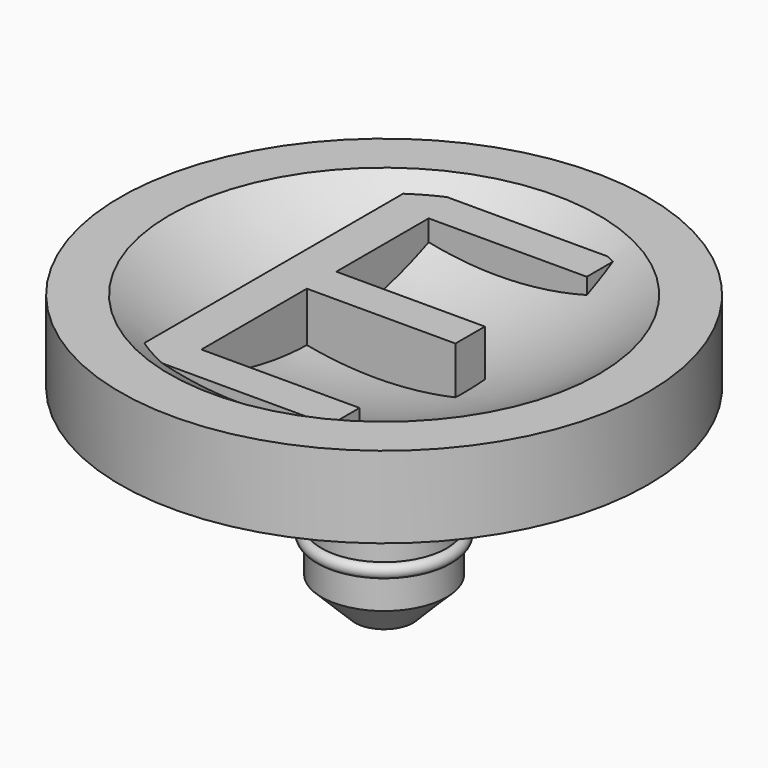
from build123d import *

# Parameters (mm, degrees)
F2_TEXT_SIZE = 19.0165314254
F3_DEPTH     = 3.4036
F4_W         = 439.3387079644
F4_H         = 117.3384692084
F5_DEPTH     = 12.7
F6_SIZE      = 1.27
F7_R         = 14.2800405429
F7_R_2       = 10
F7_R_3       = 5.842
F8_DEPTH     = 0.8
F9_SIZE      = 0.508


# Not quite as in the source:
# - Text() gives the source's letters only with a copy of the font that has no kerning and outlines rounded to 1/6400 em; it was checked with that copy


with BuildPart() as f1:
    # F0 (on Front) → F1 (revolve)
    with BuildSketch(Plane.XZ):
        with BuildLine():
            Line((2.6757909362, 0), (4.2185683136, 0))
            Line((4.2185683136, 0), (10, 0))
            Line((10, 0), (10, 5.4849551513))
            ThreePointArc((10, 5.4849551513), (5.4259986852, 2.3667937844), (0, 1.27))
            Line((0, 1.27), (0, 0))
            Line((0, 0), (0, -6.7))
            Line((0, -6.7), (2.3710267587, -6.7))
            Line((2.3710267587, -6.7), (2.3710267587, -4.308))
            ThreePointArc((2.3710267587, -4.308), (2.6250267587, -4.054), (2.3710267587, -3.8))
            Line((2.3710267587, -3.8), (2.3710267587, 0))
            Line((2.3710267587, 0), (2.6757909362, 0))
        make_face()
    revolve(axis=Axis((0, 0, 0.635), (0, 0, -1)))

    # F2 (on Top) → F3 (join)
    with BuildSketch(Plane.XY):
        with Locations((-6.0497680679, -6.806100253)):
            Text('E', F2_TEXT_SIZE, font='Open Sans', text_align=(TextAlign.LEFT, TextAlign.BOTTOM))
    extrude(amount=F3_DEPTH)

    # F4 (on Right) → F5 (cut, symmetric)
    with BuildSketch(Plane.YZ):
        with Locations((-1.8443567678, 62.5554346042)):
            Rectangle(F4_W, F4_H)
    extrude(amount=F5_DEPTH, both=True, mode=Mode.SUBTRACT)

    # F6
    f6_edges = [f1.edges().sort_by_distance(p)[0] for p in [
        (-2.371027, 0, -6.7),
    ]]
    chamfer(f6_edges, length=F6_SIZE)

    # F7 (on face) → F8 (cut)
    with BuildSketch(Plane(origin=(0, 0, 0), x_dir=(1, 0, 0), z_dir=(0, 0, -1))):
        Circle(F7_R)
        Circle(F7_R_2, mode=Mode.SUBTRACT)
        Circle(F7_R_2)
        Circle(F7_R_3, mode=Mode.SUBTRACT)
    extrude(amount=-F8_DEPTH, mode=Mode.SUBTRACT)

    # F9
    f9_edges = [f1.edges().sort_by_distance(p)[0] for p in [
        (-2.371027, 0, 0),
    ]]
    chamfer(f9_edges, length=F9_SIZE)


solid = f1.part
